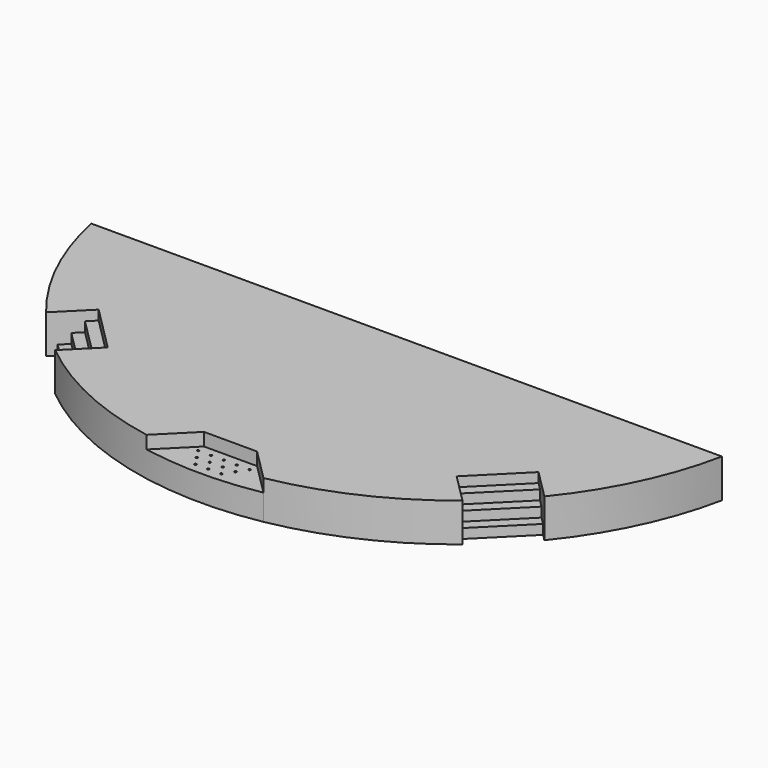
from build123d import *

# Parameters (mm, degrees)
F0_R     = 4.7625
F1_DEPTH = 914.4
F0_R_2   = 25.4
F2_DEPTH = 609.6
F3_DEPTH = 685.8
F4_DEPTH = 457.2
F5_DEPTH = 228.6


# Not quite as in the source:
# - a feature names something its author has since deleted; it is built from what else it names


with BuildPart() as f1:
    # F0 (on Top) → F1 (new body)
    with BuildSketch(Plane.XY):
        with BuildLine():
            ThreePointArc((5899.9605807424, -4822.3298462139), (6883.4780071868, -3268.3528763853), (7466.0447360031, -1524))
            Line((7466.0447360031, -1524), (-7466.0447360031, -1524))
            ThreePointArc((-7466.0447360031, -1524), (-6883.4780071868, -3268.3528763853), (-5899.9605807424, -4822.3298462139))
            Line((-5899.9605807423, -4822.329846214), (-5747.3639174843, -4669.733182956))
            Line((-5747.3639174843, -4669.733182956), (-5567.7587950629, -4490.1280605346))
            Line((-5567.7587950629, -4490.1280605346), (-5388.1536726415, -4310.5229381132))
            Line((-5388.1536726415, -4310.5229381132), (-5208.5485502201, -4130.9178156918))
            Line((-5208.5485502201, -4130.9178156918), (-4130.9178156918, -5208.5485502201))
            Line((-4130.9178156918, -5208.5485502201), (-4310.5229381132, -5388.1536726415))
            Line((-4310.5229381132, -5388.1536726415), (-4490.1280605346, -5567.7587950629))
            Line((-4490.1280605346, -5567.7587950629), (-4669.733182956, -5747.3639174843))
            Line((-4669.733182956, -5747.3639174843), (-4822.329846214, -5899.9605807423))
            ThreePointArc((-4822.3298462139, -5899.9605807424), (-3203.9850558878, -6913.6733913056), (-1384.4184602791, -7493.1826033294))
            Line((-1384.4184602791, -7493.1826033294), (-628.6179284748, -6737.3820715252))
            ThreePointArc((-628.6179284748, -6737.3820715252), (0, -6477), (628.6179284748, -6737.3820715252))
            Line((628.6179284748, -6737.3820715252), (1384.4184602791, -7493.1826033294))
            ThreePointArc((1384.4184602791, -7493.1826033294), (3203.9850558878, -6913.6733913056), (4822.3298462139, -5899.9605807424))
            Line((4822.329846214, -5899.9605807423), (4669.733182956, -5747.3639174843))
            Line((4669.733182956, -5747.3639174843), (4490.1280605346, -5567.7587950629))
            Line((4490.1280605346, -5567.7587950629), (4310.5229381132, -5388.1536726415))
            Line((4310.5229381132, -5388.1536726415), (4130.9178156918, -5208.5485502201))
            Line((4130.9178156918, -5208.5485502201), (5208.5485502201, -4130.9178156918))
            Line((5208.5485502201, -4130.9178156918), (5388.1536726415, -4310.5229381132))
            Line((5388.1536726415, -4310.5229381132), (5567.7587950629, -4490.1280605346))
            Line((5567.7587950629, -4490.1280605346), (5747.3639174843, -4669.733182956))
            Line((5747.3639174843, -4669.733182956), (5899.9605807423, -4822.329846214))
        make_face()
        with Locations((0, -5809.0438066988)):
            Circle(F0_R, mode=Mode.SUBTRACT)
        with BuildLine():
            Line((-628.6179284748, -6737.3820715252), (628.6179284748, -6737.3820715252))
            ThreePointArc((628.6179284748, -6737.3820715252), (0, -6477), (-628.6179284748, -6737.3820715252))
        make_face()
    extrude(amount=F1_DEPTH)

    # F0 (on Top) → F2 (join)
    with BuildSketch(Plane.XY):
        with BuildLine():
            Line((-628.6179284748, -6737.3820715252), (-1384.4184602791, -7493.1826033294))
            ThreePointArc((-1384.4184602791, -7493.1826033294), (-1125.4295623842, -7536.4320669739), (-865.104327551, -7570.7327586207))
            ThreePointArc((-865.104327551, -7570.7327586207), (-855.2308965756, -7123.3044838845), (-628.6179284748, -6737.3820715252))
        make_face()
        with BuildLine():
            ThreePointArc((865.104327551, -7570.7327586207), (1125.4295623842, -7536.4320669739), (1384.4184602791, -7493.1826033294))
            Line((1384.4184602791, -7493.1826033294), (628.6179284748, -6737.3820715252))
            ThreePointArc((628.6179284748, -6737.3820715252), (821.3289044025, -7025.7944286274), (889, -7366))
            ThreePointArc((889, -7366), (883.0058740441, -7469.0612749948), (865.104327551, -7570.7327586207))
        make_face()
        with BuildLine():
            ThreePointArc((-865.104327551, -7570.7327586207), (0, -7620), (865.104327551, -7570.7327586207))
            ThreePointArc((865.104327551, -7570.7327586207), (883.0058740441, -7469.0612749948), (889, -7366))
            ThreePointArc((889, -7366), (821.3289044025, -7025.7944286274), (628.6179284748, -6737.3820715252))
            Line((628.6179284748, -6737.3820715252), (-628.6179284748, -6737.3820715252))
            ThreePointArc((-628.6179284748, -6737.3820715252), (-855.2308965756, -7123.3044838845), (-865.104327551, -7570.7327586207))
        make_face()
        with Locations((-304.8, -7391.4)):
            Circle(F0_R_2, mode=Mode.SUBTRACT)
        with Locations((0, -7391.4)):
            Circle(F0_R_2, mode=Mode.SUBTRACT)
        with Locations((-457.2, -7162.8)):
            Circle(F0_R_2, mode=Mode.SUBTRACT)
        with Locations((-152.4, -7162.8)):
            Circle(F0_R_2, mode=Mode.SUBTRACT)
        with Locations((-609.6, -6934.2)):
            Circle(F0_R_2, mode=Mode.SUBTRACT)
        with Locations((-304.8, -6934.2)):
            Circle(F0_R_2, mode=Mode.SUBTRACT)
        with Locations((0, -6934.2)):
            Circle(F0_R_2, mode=Mode.SUBTRACT)
        with Locations((304.8, -7391.4)):
            Circle(F0_R_2, mode=Mode.SUBTRACT)
        with Locations((152.4, -7162.8)):
            Circle(F0_R_2, mode=Mode.SUBTRACT)
        with Locations((457.2, -7162.8)):
            Circle(F0_R_2, mode=Mode.SUBTRACT)
        with Locations((304.8, -6934.2)):
            Circle(F0_R_2, mode=Mode.SUBTRACT)
        with Locations((609.6, -6934.2)):
            Circle(F0_R_2, mode=Mode.SUBTRACT)
    extrude(amount=F2_DEPTH)

    # F0 (on Top) → F3 (join)
    with BuildSketch(Plane.XY):
        Polygon((-5208.5485502201, -4130.9178156918), (-5388.1536726415, -4310.5229381132), (-4310.5229381132, -5388.1536726415), (-4130.9178156918, -5208.5485502201), align=None)
        Polygon((4310.5229381132, -5388.1536726415), (5388.1536726415, -4310.5229381132), (5208.5485502201, -4130.9178156918), (4130.9178156918, -5208.5485502201), align=None)
    extrude(amount=F3_DEPTH)

    # F0 (on Top) → F4 (join)
    with BuildSketch(Plane.XY):
        Polygon((-5388.1536726415, -4310.5229381132), (-5567.7587950629, -4490.1280605346), (-4490.1280605346, -5567.7587950629), (-4310.5229381132, -5388.1536726415), align=None)
        Polygon((4490.1280605346, -5567.7587950629), (5567.7587950629, -4490.1280605346), (5388.1536726415, -4310.5229381132), (4310.5229381132, -5388.1536726415), align=None)
    extrude(amount=F4_DEPTH)

    # F0 (on Top) → F5 (join)
    with BuildSketch(Plane.XY):
        Polygon((-5567.7587950629, -4490.1280605346), (-5747.3639174843, -4669.733182956), (-4669.733182956, -5747.3639174843), (-4490.1280605346, -5567.7587950629), align=None)
        Polygon((4669.733182956, -5747.3639174843), (5747.3639174843, -4669.733182956), (5567.7587950629, -4490.1280605346), (4490.1280605346, -5567.7587950629), align=None)
    extrude(amount=F5_DEPTH)


solid = f1.part
